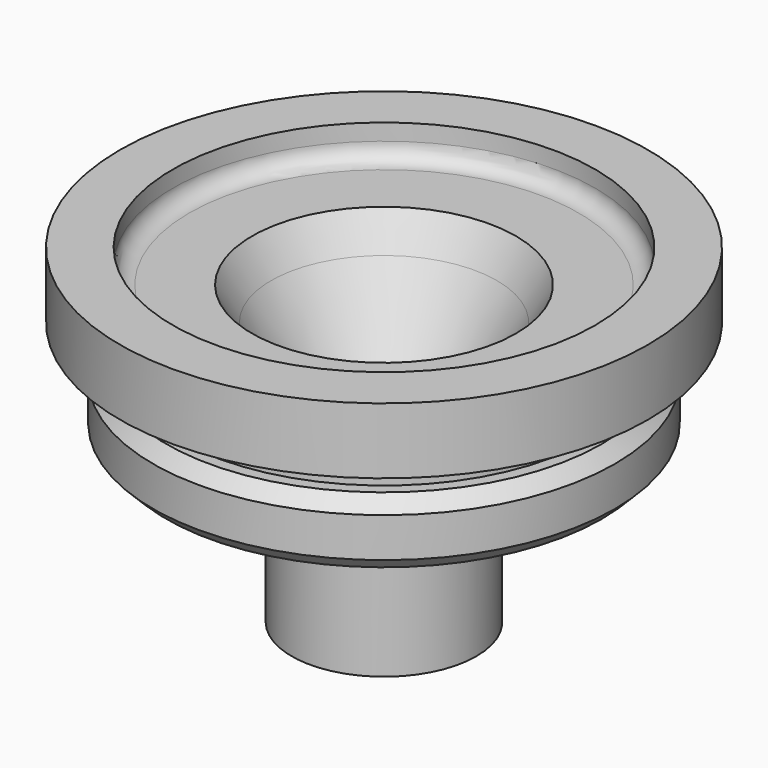
from build123d import *

# Parameters (mm, degrees)
F0_R     = 25.4
F1_DEPTH = 6.35
F4_SIZE  = 1.27
F9_R     = 1.5875


with BuildPart() as f1:
    # F0 (on Top) → F1 (new body)
    with BuildSketch(Plane.XY):
        Circle(F0_R)
    extrude(amount=-F1_DEPTH)

    # F2 (on Front) → F3 (revolve)
    with BuildSketch(Plane.XZ):
        Polygon((19.85, -6.35), (0, -6.35), (0, -31.75), (9.525, -31.75), (9.525, -16.2), (22.225, -16.2), (22.225, -9.85), (19.85, -9.85), align=None)
    revolve(axis=Axis((0, 0, -19.05), (0, 0, 1)))

    # F4
    f4_edges = [f1.edges().sort_by_distance(p)[0] for p in [
        (-22.225, 0, -9.85),
        (-22.225, 0, -16.2),
    ]]
    chamfer(f4_edges, length=F4_SIZE)

    # F5 (on Front) → F6 (revolve, cut)
    with BuildSketch(Plane.XZ):
        Polygon((20.32, 0), (0, 0), (0, -6.35), (10.8669128953, -6.35), (12.7, -3.175), (20.32, -3.175), align=None)
        Polygon((10.8669128953, -6.35), (0, -6.35), (0, -42.1200841665), (6.35, -42.1200841665), (6.35, -14.1735226281), align=None)
    revolve(axis=Axis((0, 0, 5.083523225), (0, 0, 1)), mode=Mode.SUBTRACT)

    # F7 (on Front) → F8 (revolve, cut)
    with BuildSketch(Plane.XZ):
        Polygon((16.51, -31.75), (16.51, -16.2), (9.525, -16.2), (8.89, -16.2), (8.89, -31.75), (9.525, -31.75), align=None)
        Polygon((9.525, -16.2), (16.51, -16.2), (16.51, -6.675), (13.6122134253, -6.675), (8.89, -14.8541135768), (8.89, -16.2), align=None)
    revolve(axis=Axis((0, 0, -10.6237775408), (0, 0, 1)), mode=Mode.SUBTRACT)

    # F9
    f9_edges = [f1.edges().sort_by_distance(p)[0] for p in [
        (-16.51, 0, -6.675),
        (16.51, 0, -11.4375),
        (-13.612213, 0, -6.675),
        (-20.32, 0, -3.175),
        (-8.89, 0, -14.854114),
    ]]
    fillet(f9_edges, radius=F9_R)


solid = f1.part
